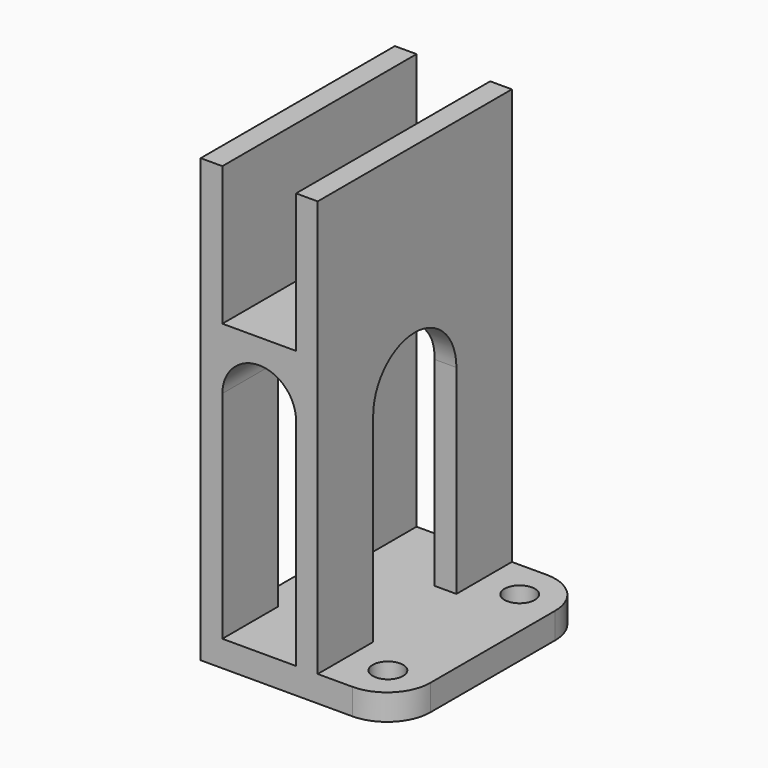
from build123d import *

# Parameters (mm, degrees)
F1_DEPTH     = 28
F2_R         = 1.75
F3_DEPTH     = 25
F4_W         = 12
F4_H         = 29
F5_DEPTH     = 25
F6_T4_DEPTH  = 28
F6_T10_DEPTH = 28
F6_T16_DEPTH = 28
F6_T23_DEPTH = 28
F6_T29_DEPTH = 28
F6_T35_DEPTH = 28
F6_T41_DEPTH = 28
F6_T47_DEPTH = 28
F6_T54_DEPTH = 28
F6_T60_DEPTH = 28
F7_R         = 5.99999
F8_R         = 5


# Not quite as in the source:
# - a fillet or chamfer that OpenCascade refuses, or shapes differently, is made with other operations: its cross-section is extruded or revolved along the edge and cut away or added
# - a fillet or chamfer is up to 0.001 mm smaller than in the source, because OpenCascade refuses the exact size


with BuildPart() as f1:
    # F0 (on Front) → F1 (new body)
    with BuildSketch(Plane.XZ):
        Polygon((-4.25, 25.5), (-6.75, 25.5), (-6.75, -22.5), (-6.75, -25.5), (-4.25, -25.5), (4.25, -25.5), (6.75, -25.5), (15.75, -25.5), (15.75, -22.5), (6.75, -22.5), (6.75, 25.5), (4.25, 25.5), (4.25, 9.5), (0, 9.5), (-4.25, 9.5), align=None)
        Polygon((4.25, -22.5), (-4.25, -22.5), (-4.25, 6.6576944664), (0, 6.6576944664), (4.25, 6.6576944664), align=None, mode=Mode.SUBTRACT)
    extrude(amount=F1_DEPTH)

    # F2 (on face) → F3 (cut)
    with BuildSketch(Plane(origin=(0, 0, -25.5), x_dir=(1, 0, 0), z_dir=(0, 0, -1))):
        with Locations((11.25, 23.5)):
            Circle(F2_R)
        with Locations((11.25, 4.5)):
            Circle(F2_R)
    extrude(amount=-F3_DEPTH, mode=Mode.SUBTRACT)

    # F4 (on face) → F5 (cut)
    with BuildSketch(Plane.YZ.offset(6.75)):
        with Locations((-14, -8)):
            Rectangle(F4_W, F4_H)
    extrude(amount=-F5_DEPTH, mode=Mode.SUBTRACT)

    # F6: fillet of radius 4.25 on 2 edges, made by hand


with BuildPart() as f6_tool2:
    # F6_s3 → F6_t4 (new body)
    with BuildSketch(Plane.XZ):
        with BuildLine():
            ThreePointArc((0, 6.6576944664), (3.00520382, 5.4128982865), (4.25, 2.4076944664))
            Line((4.25, 2.4076944664), (4.25, 6.6576944664))
            Line((4.25, 6.6576944664), (0, 6.6576944664))
        make_face()
    extrude(amount=F6_T4_DEPTH)

    split(bisect_by=Plane.XZ.offset(8), keep=Keep.BOTTOM)

    split(bisect_by=Plane.XY.offset(6.5), keep=Keep.TOP)


with BuildPart() as f1_1:
    add(f1.part)

    # F6_t1: union F6_tool2
    add(f6_tool2.part)


with BuildPart() as f6_tool8:
    # F6_s9 → F6_t10 (new body)
    with BuildSketch(Plane.XZ):
        with BuildLine():
            ThreePointArc((0, 6.6576944664), (3.00520382, 5.4128982865), (4.25, 2.4076944664))
            Line((4.25, 2.4076944664), (4.25, 6.6576944664))
            Line((4.25, 6.6576944664), (0, 6.6576944664))
        make_face()
    extrude(amount=F6_T10_DEPTH)

    split(bisect_by=Plane.XZ.offset(8), keep=Keep.BOTTOM)

    split(bisect_by=Plane.XY.offset(6.5), keep=Keep.BOTTOM)


with BuildPart() as f1_2:
    add(f1_1.part)

    # F6_t7: union F6_tool8
    add(f6_tool8.part)


with BuildPart() as f6_tool14:
    # F6_s15 → F6_t16 (new body)
    with BuildSketch(Plane.XZ):
        with BuildLine():
            ThreePointArc((0, 6.6576944664), (3.00520382, 5.4128982865), (4.25, 2.4076944664))
            Line((4.25, 2.4076944664), (4.25, 6.6576944664))
            Line((4.25, 6.6576944664), (0, 6.6576944664))
        make_face()
    extrude(amount=F6_T16_DEPTH)

    split(bisect_by=Plane.XZ.offset(8), keep=Keep.TOP)

    split(bisect_by=Plane.XY.offset(6.5), keep=Keep.TOP)

    split(bisect_by=Plane.XZ.offset(20), keep=Keep.BOTTOM)


with BuildPart() as f1_3:
    add(f1_2.part)

    # F6_t13: union F6_tool14
    add(f6_tool14.part)


with BuildPart() as f6_tool21:
    # F6_s22 → F6_t23 (new body)
    with BuildSketch(Plane.XZ):
        with BuildLine():
            ThreePointArc((0, 6.6576944664), (3.00520382, 5.4128982865), (4.25, 2.4076944664))
            Line((4.25, 2.4076944664), (4.25, 6.6576944664))
            Line((4.25, 6.6576944664), (0, 6.6576944664))
        make_face()
    extrude(amount=F6_T23_DEPTH)

    split(bisect_by=Plane.XY.offset(6.5), keep=Keep.TOP)

    split(bisect_by=Plane.XZ.offset(20), keep=Keep.TOP)


with BuildPart() as f1_4:
    add(f1_3.part)

    # F6_t20: union F6_tool21
    add(f6_tool21.part)


with BuildPart() as f6_tool27:
    # F6_s28 → F6_t29 (new body)
    with BuildSketch(Plane.XZ):
        with BuildLine():
            ThreePointArc((0, 6.6576944664), (3.00520382, 5.4128982865), (4.25, 2.4076944664))
            Line((4.25, 2.4076944664), (4.25, 6.6576944664))
            Line((4.25, 6.6576944664), (0, 6.6576944664))
        make_face()
    extrude(amount=F6_T29_DEPTH)

    split(bisect_by=Plane.XY.offset(6.5), keep=Keep.BOTTOM)

    split(bisect_by=Plane.XZ.offset(20), keep=Keep.TOP)


with BuildPart() as f1_5:
    add(f1_4.part)

    # F6_t26: union F6_tool27
    add(f6_tool27.part)


with BuildPart() as f6_tool33:
    # F6_s34 → F6_t35 (new body)
    with BuildSketch(Plane.XZ):
        with BuildLine():
            ThreePointArc((-4.25, 2.4076944664), (-3.00520382, 5.4128982865), (0, 6.6576944664))
            Line((0, 6.6576944664), (-4.25, 6.6576944664))
            Line((-4.25, 6.6576944664), (-4.25, 2.4076944664))
        make_face()
    extrude(amount=F6_T35_DEPTH)

    split(bisect_by=Plane.XZ.offset(8), keep=Keep.BOTTOM)

    split(bisect_by=Plane.XY.offset(6.5), keep=Keep.BOTTOM)


with BuildPart() as f1_6:
    add(f1_5.part)

    # F6_t32: union F6_tool33
    add(f6_tool33.part)


with BuildPart() as f6_tool39:
    # F6_s40 → F6_t41 (new body)
    with BuildSketch(Plane.XZ):
        with BuildLine():
            ThreePointArc((-4.25, 2.4076944664), (-3.00520382, 5.4128982865), (0, 6.6576944664))
            Line((0, 6.6576944664), (-4.25, 6.6576944664))
            Line((-4.25, 6.6576944664), (-4.25, 2.4076944664))
        make_face()
    extrude(amount=F6_T41_DEPTH)

    split(bisect_by=Plane.XZ.offset(8), keep=Keep.BOTTOM)

    split(bisect_by=Plane.XY.offset(6.5), keep=Keep.TOP)


with BuildPart() as f1_7:
    add(f1_6.part)

    # F6_t38: union F6_tool39
    add(f6_tool39.part)


with BuildPart() as f6_tool45:
    # F6_s46 → F6_t47 (new body)
    with BuildSketch(Plane.XZ):
        with BuildLine():
            ThreePointArc((-4.25, 2.4076944664), (-3.00520382, 5.4128982865), (0, 6.6576944664))
            Line((0, 6.6576944664), (-4.25, 6.6576944664))
            Line((-4.25, 6.6576944664), (-4.25, 2.4076944664))
        make_face()
    extrude(amount=F6_T47_DEPTH)

    split(bisect_by=Plane.XZ.offset(20), keep=Keep.BOTTOM)

    split(bisect_by=Plane.XZ.offset(8), keep=Keep.TOP)

    split(bisect_by=Plane.XY.offset(6.5), keep=Keep.TOP)


with BuildPart() as f1_8:
    add(f1_7.part)

    # F6_t44: union F6_tool45
    add(f6_tool45.part)


with BuildPart() as f6_tool52:
    # F6_s53 → F6_t54 (new body)
    with BuildSketch(Plane.XZ):
        with BuildLine():
            ThreePointArc((-4.25, 2.4076944664), (-3.00520382, 5.4128982865), (0, 6.6576944664))
            Line((0, 6.6576944664), (-4.25, 6.6576944664))
            Line((-4.25, 6.6576944664), (-4.25, 2.4076944664))
        make_face()
    extrude(amount=F6_T54_DEPTH)

    split(bisect_by=Plane.XZ.offset(20), keep=Keep.TOP)

    split(bisect_by=Plane.XY.offset(6.5), keep=Keep.BOTTOM)


with BuildPart() as f1_9:
    add(f1_8.part)

    # F6_t51: union F6_tool52
    add(f6_tool52.part)


with BuildPart() as f6_tool58:
    # F6_s59 → F6_t60 (new body)
    with BuildSketch(Plane.XZ):
        with BuildLine():
            ThreePointArc((-4.25, 2.4076944664), (-3.00520382, 5.4128982865), (0, 6.6576944664))
            Line((0, 6.6576944664), (-4.25, 6.6576944664))
            Line((-4.25, 6.6576944664), (-4.25, 2.4076944664))
        make_face()
    extrude(amount=F6_T60_DEPTH)

    split(bisect_by=Plane.XZ.offset(20), keep=Keep.TOP)

    split(bisect_by=Plane.XY.offset(6.5), keep=Keep.TOP)


with BuildPart() as f1_10:
    add(f1_9.part)

    # F6_t57: union F6_tool58
    add(f6_tool58.part)

    # F7 (radius 6 in the source; OpenCascade refuses exactly that, so slightly less here)
    f7_edges = [f1_10.edges().sort_by_distance(p)[0] for p in [
        (3.948484, -20, 6.5),
        (-3.948484, -20, 6.5),
        (-3.948484, -8, 6.5),
        (3.948484, -8, 6.5),
    ]]
    fillet(f7_edges, radius=F7_R)

    # F8
    f8_edges = [f1_10.edges().sort_by_distance(p)[0] for p in [
        (15.75, 0, -24),
        (15.75, -28, -24),
    ]]
    fillet(f8_edges, radius=F8_R)


solid = f1_10.part
